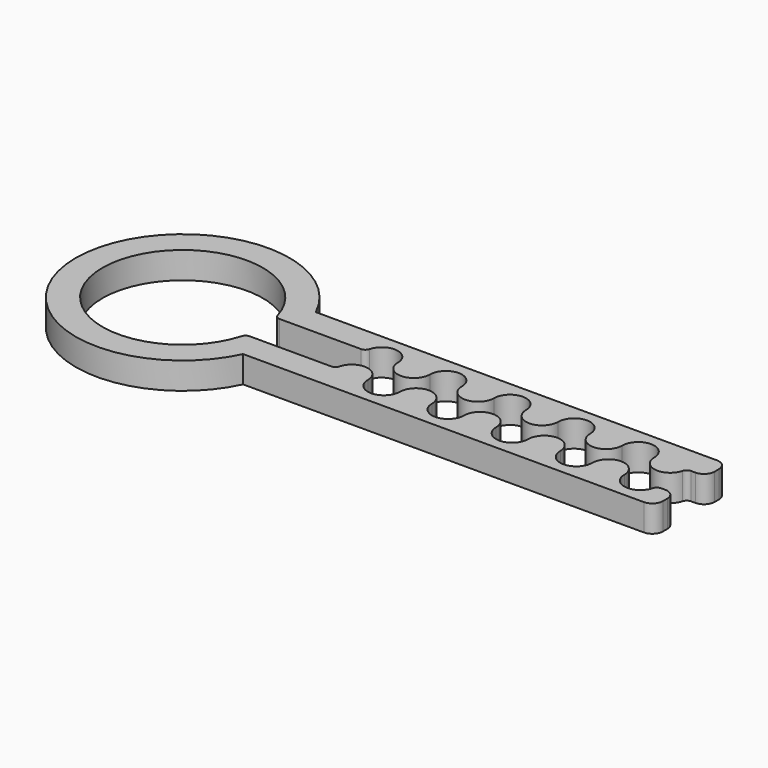
from build123d import *

# Parameters (mm, degrees)
F1_DEPTH = 5
F2_R     = 1


with BuildPart() as f1:
    # F0 (on Top) → F1 (new body)
    with BuildSketch(Plane.XY):
        with BuildLine():
            ThreePointArc((-38.5927113062, 7.2194887325), (-35.5927113062, 10.2194887325), (-32.5927113062, 7.2194887325))
            ThreePointArc((-32.5927113062, 7.2194887325), (-29.5927113062, 4.2194887325), (-26.5927113062, 7.2194887325))
            ThreePointArc((-26.5927113062, 7.2194887325), (-23.5927113062, 10.2194887325), (-20.5927113062, 7.2194887325))
            ThreePointArc((-20.5927113062, 7.2194887325), (-17.5927113062, 4.2194887325), (-14.5927113062, 7.2194887325))
            ThreePointArc((-14.5927113062, 7.2194887325), (-11.5927113062, 10.2194887325), (-8.5927113062, 7.2194887325))
            ThreePointArc((-8.5927113062, 7.2194887325), (-5.5927113062, 4.2194887325), (-2.5927113062, 7.2194887325))
            ThreePointArc((-2.5927113062, 7.2194887325), (0.4072886938, 10.2194887325), (3.4072886938, 7.2194887325))
            ThreePointArc((3.4072886938, 7.2194887325), (6.4072886938, 4.2194887325), (9.4072886938, 7.2194887325))
            ThreePointArc((9.4072886938, 7.2194887325), (12.4072886938, 10.2194887325), (15.4072886938, 7.2194887325))
            ThreePointArc((15.4072886938, 7.2194887325), (18.4072886938, 4.2194887325), (21.4072886938, 7.2194887325))
            Line((21.4072886938, 7.2194887325), (23.1027154343, 7.2194887325))
            ThreePointArc((23.1027154343, 7.2194887325), (24.5169289967, 7.8052751701), (25.1027154343, 9.2194887325))
            Line((25.1027154343, 9.2194887325), (25.1027154343, 10.2194887325))
            ThreePointArc((25.1027154343, 10.2194887325), (24.5169289967, 11.6337022949), (23.1027154343, 12.2194887325))
            Line((23.1027154343, 12.2194887325), (-51.9450229577, 12.2194887325))
            ThreePointArc((-51.9450229577, 12.2194887325), (-90.0488899479, 3.7194887325), (-51.9450229577, -4.7805112675))
            Line((-51.9450229577, -4.7805112675), (23.0392886417, -4.7805112675))
            ThreePointArc((23.0392886417, -4.7805112675), (24.4535022041, -4.1947248299), (25.0392886417, -2.7805112675))
            Line((25.0392886417, -2.7805112675), (25.0392886417, -1.7805112675))
            ThreePointArc((25.0392886417, -1.7805112675), (24.4535022041, -0.3662977051), (23.0392886417, 0.2194887325))
            Line((23.0392886417, 0.2194887325), (21.4072886938, 0.2194887325))
            ThreePointArc((21.4072886938, 0.2194887325), (18.4072886938, -2.7805112675), (15.4072886938, 0.2194887325))
            ThreePointArc((15.4072886938, 0.2194887325), (12.4072886938, 3.2194887325), (9.4072886938, 0.2194887325))
            ThreePointArc((9.4072886938, 0.2194887325), (6.4072886938, -2.7805112675), (3.4072886938, 0.2194887325))
            ThreePointArc((3.4072886938, 0.2194887325), (0.4072886938, 3.2194887325), (-2.5927113062, 0.2194887325))
            ThreePointArc((-2.5927113062, 0.2194887325), (-5.5927113062, -2.7805112675), (-8.5927113062, 0.2194887325))
            ThreePointArc((-8.5927113062, 0.2194887325), (-11.5927113062, 3.2194887325), (-14.5927113062, 0.2194887325))
            ThreePointArc((-14.5927113062, 0.2194887325), (-17.5927113062, -2.7805112675), (-20.5927113062, 0.2194887325))
            ThreePointArc((-20.5927113062, 0.2194887325), (-23.5927113062, 3.2194887325), (-26.5927113062, 0.2194887325))
            ThreePointArc((-26.5927113062, 0.2194887325), (-29.5927113062, -2.7805112675), (-32.5927113062, 0.2194887325))
            ThreePointArc((-32.5927113062, 0.2194887325), (-35.5927113062, 3.2194887325), (-38.5927113062, 0.2194887325))
            Line((-38.5927113062, 0.2194887325), (-55.4629378021, 0.2194887325))
            ThreePointArc((-55.4629378021, 0.2194887325), (-85.0488899479, 3.7194887325), (-55.4629378021, 7.2194887325))
            Line((-55.4629378021, 7.2194887325), (-38.5927113062, 7.2194887325))
        make_face()
    extrude(amount=F1_DEPTH)

    # F2
    f2_edges = [f1.edges().sort_by_distance(p)[0] for p in [
        (-55.462938, 7.219489, 2.5),
        (-38.592711, 7.219489, 2.5),
        (-38.592711, 0.219489, 2.5),
        (-55.462938, 0.219489, 2.5),
        (21.407289, 0.219489, 2.5),
        (21.407289, 7.219489, 2.5),
    ]]
    fillet(f2_edges, radius=F2_R)


solid = f1.part
